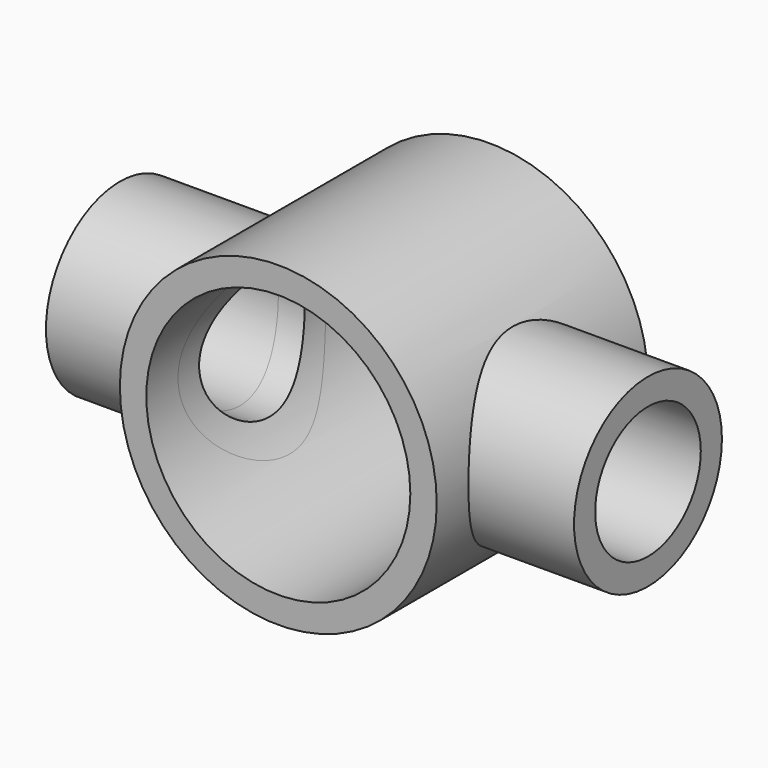
from build123d import *
from build123d import SkipClean  # not in build123d's __all__

# Parameters (mm, degrees)
F0_R          = 30
F0_R_2        = 25
F1_DEPTH      = 25
F1_DEPTH_BACK = 25
F2_R          = 17.5
F2_R_2        = 12.5
F3_DEPTH      = 50
F3_DEPTH_BACK = 50
F4_R          = 25
F5_DEPTH      = 50
F6_R          = 12.5
F7_DEPTH      = 100.0010001


with BuildPart() as f1:
    # F0 (on Front) → F1 (new body, two sides)
    with BuildSketch(Plane.XZ) as f1_sk:
        Circle(F0_R)
        Circle(F0_R_2, mode=Mode.SUBTRACT)
    extrude(amount=F1_DEPTH)
    extrude(f1_sk.sketch, amount=-F1_DEPTH_BACK)

    # F2 (on Right) → F3 (join, two sides)
    with BuildSketch(Plane.YZ) as f3_sk:
        Circle(F2_R)
        Circle(F2_R_2, mode=Mode.SUBTRACT)
    extrude(amount=F3_DEPTH)
    extrude(f3_sk.sketch, amount=-F3_DEPTH_BACK)

    # F4 (on face) → F5 (cut, through all)
    with BuildSketch(Plane.XZ.offset(25)):
        Circle(F4_R)
    extrude(amount=-F5_DEPTH, mode=Mode.SUBTRACT)

    # F6 (on face) → F7 (cut, through all)
    with BuildSketch(Plane.YZ.offset(50)):
        Circle(F6_R)
    with SkipClean():  # cleaning this boolean's faces spoils the solid; the shape is the same uncleaned
        extrude(amount=-F7_DEPTH, mode=Mode.SUBTRACT)


solid = f1.part
